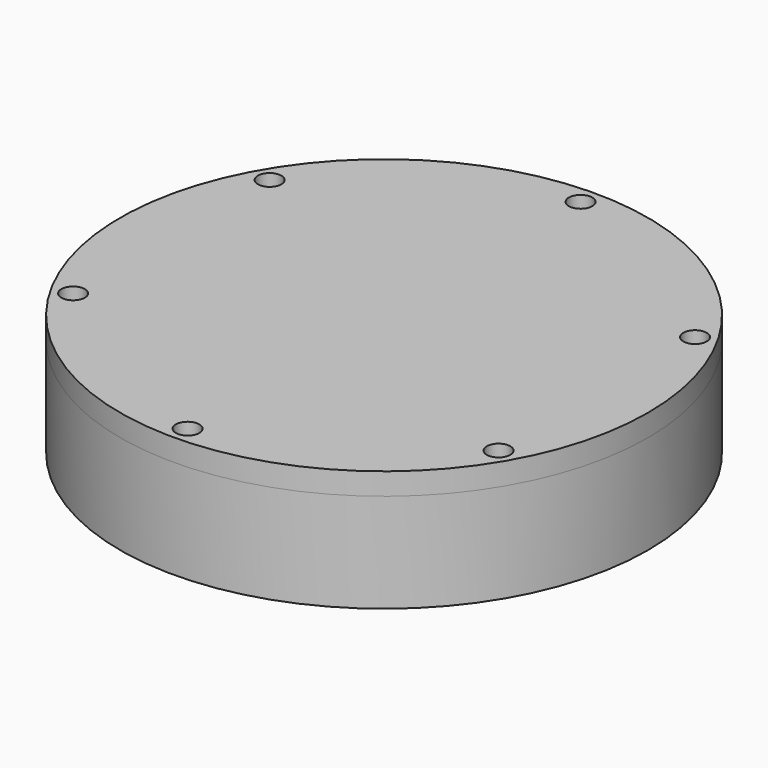
from build123d import *

# Parameters (mm, degrees)
F0_R      = 4.9
F1_DEPTH  = 7.5
F2_R      = 17.5
F3_DEPTH  = 7.5
F4_R      = 36
F4_R_2    = 31
F4_R_3    = 4.9
F5_DEPTH  = 3
F6_DEPTH  = 7.5
F7_R      = 36
F7_R_2    = 31
F8_DEPTH  = 3
F10_DEPTH = 3
F11_R     = 36
F11_R_2   = 2.35
F12_DEPTH = 3
F13_R     = 1.6
F14_DEPTH = 25
F15_DEPTH = 25


# Not quite as in the source:
# - a pattern or mirror of a feature is missing from the dataset's text; its kind, count and spacing are read off the source's solid


with BuildPart() as f1:
    # F0 (on Top) → F1 (new body)
    with BuildSketch(Plane.XY):
        with BuildLine():
            ThreePointArc((11.0418925329, 5.1091726771), (5.0196860546, 6.909005132), (1.4469795247, 12.08028503))
            ThreePointArc((1.4469795247, 12.08028503), (0, 13.185), (-1.4469795247, 12.08028503))
            ThreePointArc((-1.4469795247, 12.08028503), (-5.0196860546, 6.909005132), (-11.0418925329, 5.1091726771))
            ThreePointArc((-11.0418925329, 5.1091726771), (-12.5396801674, 4.0743890708), (-11.9361750602, 2.3568540652))
            ThreePointArc((-11.9361750602, 2.3568540652), (-8.1220226492, -2.639005132), (-8.2712444102, -8.9226426612))
            ThreePointArc((-8.2712444102, -8.9226426612), (-7.7499485515, -10.6668890708), (-5.9299823581, -10.6236691112))
            ThreePointArc((-5.9299823581, -10.6236691112), (0, -8.54), (5.9299823581, -10.6236691112))
            ThreePointArc((5.9299823581, -10.6236691112), (7.7499485515, -10.6668890708), (8.2712444102, -8.9226426612))
            ThreePointArc((8.2712444102, -8.9226426612), (8.1220226492, -2.639005132), (11.9361750602, 2.3568540652))
            ThreePointArc((11.9361750602, 2.3568540652), (12.5396801674, 4.0743890708), (11.0418925329, 5.1091726771))
        make_face()
        Circle(F0_R, mode=Mode.SUBTRACT)
    extrude(amount=F1_DEPTH)


with BuildPart() as f3:
    # F2 (on Top) → F3 (new body)
    with BuildSketch(Plane.XY):
        with Locations((0, -2.4335)):
            Circle(F2_R)
        with BuildLine():
            ThreePointArc((-1.4782610314, 12.8194490581), (0, 14.065), (1.4782610314, 12.8194490581))
            ThreePointArc((1.4782610314, 12.8194490581), (5.48675, 7.0698297684), (12.4703108513, 6.4731861356))
            ThreePointArc((12.4703108513, 6.4731861356), (14.2881201243, 5.81575), (13.9485718827, 3.9127629225))
            ThreePointArc((13.9485718827, 3.9127629225), (10.9735, -2.4335), (13.9485718827, -8.7797629225))
            ThreePointArc((13.9485718827, -8.7797629225), (14.2881201243, -10.68275), (12.4703108513, -11.3401861356))
            ThreePointArc((12.4703108513, -11.3401861356), (5.48675, -11.9368297684), (1.4782610314, -17.6864490581))
            ThreePointArc((1.4782610314, -17.6864490581), (0, -18.932), (-1.4782610314, -17.6864490581))
            ThreePointArc((-1.4782610314, -17.6864490581), (-5.48675, -11.9368297684), (-12.4703108513, -11.3401861356))
            ThreePointArc((-12.4703108513, -11.3401861356), (-14.2881201243, -10.68275), (-13.9485718827, -8.7797629225))
            ThreePointArc((-13.9485718827, -8.7797629225), (-10.9735, -2.4335), (-13.9485718827, 3.9127629225))
            ThreePointArc((-13.9485718827, 3.9127629225), (-14.2881201243, 5.81575), (-12.4703108513, 6.4731861356))
            ThreePointArc((-12.4703108513, 6.4731861356), (-5.48675, 7.0698297684), (-1.4782610314, 12.8194490581))
        make_face(mode=Mode.SUBTRACT)
    extrude(amount=F3_DEPTH)


with BuildPart() as f5:
    # F4 (on Top) → F5 (new body)
    with BuildSketch(Plane.XY):
        with Locations((0, -2.4335)):
            Circle(F4_R)
        with Locations((0, -2.4335)):
            Circle(F4_R_2, mode=Mode.SUBTRACT)
        with Locations((0, -2.4335)):
            Circle(F4_R_2)
        Circle(F4_R_3, mode=Mode.SUBTRACT)
    extrude(amount=-F5_DEPTH)

    # F4 (on Top) → F6 (join)
    with BuildSketch(Plane.XY):
        with Locations((0, -2.4335)):
            Circle(F4_R)
        with Locations((0, -2.4335)):
            Circle(F4_R_2, mode=Mode.SUBTRACT)
    extrude(amount=F6_DEPTH)

    # F9 (on face) → F10 (cut, through all)
    with BuildSketch(Plane(origin=(0, 0, -3), x_dir=(1, 0, 0), z_dir=(0, 0, -1))):
        with BuildLine():
            ThreePointArc((10.1448459521, 10.6049030387), (7.1680744716, 10.5389029721), (7.2340745381, 7.5621314916))
            ThreePointArc((7.2340745381, 7.5621314916), (10.4650689018, 0), (7.2340745381, -7.5621314916))
            ThreePointArc((7.2340745381, -7.5621314916), (7.1680744716, -10.5389029721), (10.1448459521, -10.6049030387))
            ThreePointArc((10.1448459521, -10.6049030387), (14.6758941074, 0), (10.1448459521, 10.6049030387))
        make_face()
    f10 = extrude(amount=-F10_DEPTH, mode=Mode.SUBTRACT)

    # F10_copies: F10 across plane
    add(f10.mirror(Plane(origin=(0, 0, 0), x_dir=(0, 0, -1), z_dir=(-1, 0, 0))), mode=Mode.SUBTRACT)

    # F11 (on face) → F12 (join)
    with BuildSketch(Plane(origin=(0, 0, -3), x_dir=(1, 0, 0), z_dir=(0, 0, -1))):
        with Locations((0, 2.4335)):
            Circle(F11_R)
        with Locations((-8.6894602451, 9.0835172651)):
            Circle(F11_R_2, mode=Mode.SUBTRACT)
        with Locations((8.6894602451, 9.0835172651)):
            Circle(F11_R_2, mode=Mode.SUBTRACT)
    extrude(amount=F12_DEPTH)


with BuildPart() as f8:
    # F7 (on face) → F8 (new body)
    with BuildSketch(Plane.XY.offset(7.5)):
        with Locations((0, -2.4335)):
            Circle(F7_R)
        with Locations((0, -2.4335)):
            Circle(F7_R_2, mode=Mode.SUBTRACT)
        with Locations((0, -2.4335)):
            Circle(F7_R_2)
    extrude(amount=F8_DEPTH)


with BuildPart() as f14_tool:
    # F13 (on face) → F14 (new body)
    with BuildSketch(Plane.XY.offset(10.5)):
        with Locations((0, 31.0665)):
            Circle(F13_R)
        with Locations((-29.0118510268, 14.3165)):
            Circle(F13_R)
        with Locations((-29.0118510268, -19.1835)):
            Circle(F13_R)
        with Locations((0, -35.9335)):
            Circle(F13_R)
        with Locations((29.0118510268, -19.1835)):
            Circle(F13_R)
        with Locations((29.0118510268, 14.3165)):
            Circle(F13_R)
    extrude(amount=-F14_DEPTH)


with BuildPart() as f5_1:
    add(f5.part)

    # F14: cut by f14_tool
    add(f14_tool.part, mode=Mode.SUBTRACT)

    # F0 (on Top) → F15 (cut)
    with BuildSketch(Plane.XY):
        Circle(F0_R)
    extrude(amount=-F15_DEPTH, mode=Mode.SUBTRACT)


with BuildPart() as f8_1:
    add(f8.part)

    # F14: cut by f14_tool
    add(f14_tool.part, mode=Mode.SUBTRACT)


solid = Compound([f1.part, f3.part, f5_1.part, f8_1.part])
